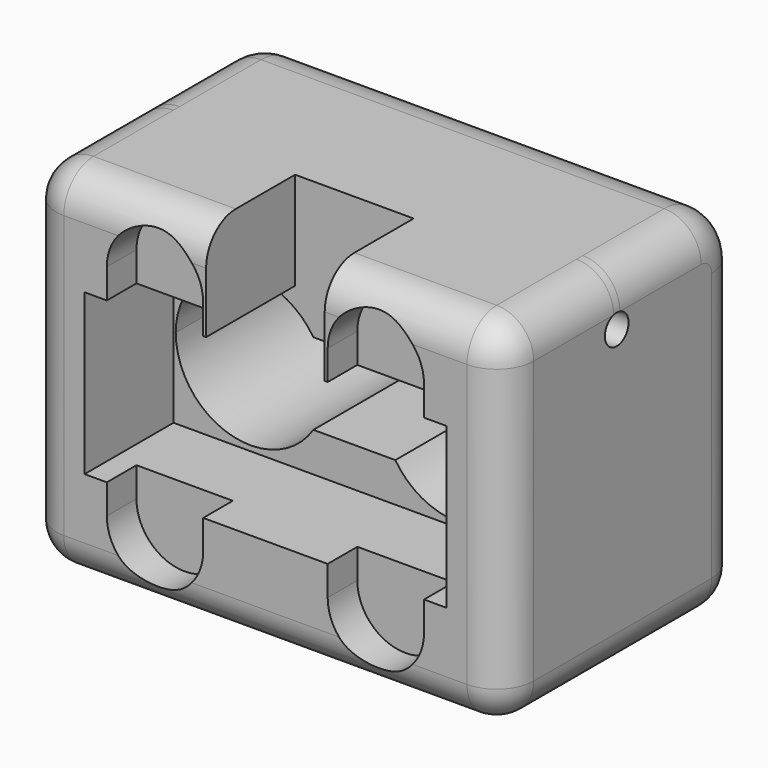
from build123d import *

# Parameters (mm, degrees)
F1_DEPTH      = 5
F3_DEPTH      = 10
F5_DEPTH      = 25
F7_R          = 6.7597979746
F6_R          = 2
F8_DEPTH      = 69.4
F9_R          = 5
F10_R         = 5
F11_T1_DEPTH  = 44.2
F11_T3_DEPTH  = 44.2
F12_T1_DEPTH  = 54.4
F12_T3_DEPTH  = 30
F12_T5_DEPTH  = 38
F12_S9_W      = 5
F12_S9_H      = 5
F12_T10_DEPTH = 5
F12_S15_W     = 5
F12_S15_H     = 5
F12_T16_DEPTH = 5
F12_S21_W     = 5
F12_S21_H     = 5
F12_T22_DEPTH = 5
F12_S27_W     = 5
F12_S27_H     = 5
F12_T28_DEPTH = 5
F12_T32_ANGLE = 90
F12_T34_ANGLE = 90


# Not quite as in the source:
# - a fillet or chamfer that OpenCascade refuses, or shapes differently, is made with other operations: its cross-section is extruded or revolved along the edge and cut away or added


with BuildPart() as f1:
    # F0 (on Front) → F1 (new body)
    with BuildSketch(Plane.XZ):
        with BuildLine():
            Line((32.2, -24), (32.2, 24))
            Line((32.2, 24), (8, 24))
            Line((8, 24), (8, 10.8))
            Line((8, 10.8), (8.4, 10.8))
            Line((8.4, 10.8), (8.4, 14.8))
            ThreePointArc((8.4, 14.8), (14.9, 21.3), (21.4, 14.8))
            Line((21.4, 14.8), (21.4, 10.8))
            Line((21.4, 10.8), (24.4, 10.8))
            Line((24.4, 10.8), (24.4, -10.8))
            Line((24.4, -10.8), (21.4, -10.8))
            Line((21.4, -10.8), (21.4, -14.8))
            ThreePointArc((21.4, -14.8), (14.9, -21.3), (8.4, -14.8))
            Line((8.4, -14.8), (8.4, -10.8))
            Line((8.4, -10.8), (-8.4, -10.8))
            Line((-8.4, -10.8), (-8.4, -14.8))
            ThreePointArc((-8.4, -14.8), (-14.9, -21.3), (-21.4, -14.8))
            Line((-21.4, -14.8), (-21.4, -10.8))
            Line((-21.4, -10.8), (-24.4, -10.8))
            Line((-24.4, -10.8), (-24.4, 10.8))
            Line((-24.4, 10.8), (-21.4, 10.8))
            Line((-21.4, 10.8), (-21.4, 14.8))
            ThreePointArc((-21.4, 14.8), (-14.9, 21.3), (-8.4, 14.8))
            Line((-8.4, 14.8), (-8.4, 10.8))
            Line((-8.4, 10.8), (-8, 10.8))
            Line((-8, 10.8), (-8, 24))
            Line((-8, 24), (-32.2, 24))
            Line((-32.2, 24), (-32.2, -24))
            Line((-32.2, -24), (32.2, -24))
        make_face()
    extrude(amount=F1_DEPTH)

    # F2 (on face) → F3 (join)
    with BuildSketch(Plane(origin=(0, 0, 0), x_dir=(-1, 0, 0), z_dir=(0, 1, 0))):
        with BuildLine():
            Line((24.4, 10.8), (24.4, -10.8))
            Line((24.4, -10.8), (21.4, -10.8))
            Line((21.4, -10.8), (21.4, -14.8))
            ThreePointArc((21.4, -14.8), (14.9, -21.3), (8.4, -14.8))
            Line((8.4, -14.8), (8.4, -10.8))
            Line((8.4, -10.8), (-8.4, -10.8))
            Line((-8.4, -10.8), (-8.4, -14.8))
            ThreePointArc((-8.4, -14.8), (-14.9, -21.3), (-21.4, -14.8))
            Line((-21.4, -14.8), (-21.4, -10.8))
            Line((-21.4, -10.8), (-24.4, -10.8))
            Line((-24.4, -10.8), (-24.4, 10.8))
            Line((-24.4, 10.8), (-21.4, 10.8))
            Line((-21.4, 10.8), (-21.4, 14.8))
            ThreePointArc((-21.4, 14.8), (-14.9, 21.3), (-8.4, 14.8))
            Line((-8.4, 14.8), (-8.4, 10.8))
            Line((-8.4, 10.8), (-8, 10.8))
            Line((-8, 10.8), (-8, 24))
            Line((-8, 24), (-32.2, 24))
            Line((-32.2, 24), (-32.2, -24))
            Line((-32.2, -24), (32.2, -24))
            Line((32.2, -24), (32.2, 24))
            Line((32.2, 24), (8, 24))
            Line((8, 24), (8, 10.8))
            Line((8, 10.8), (8.4, 10.8))
            Line((8.4, 10.8), (8.4, 14.8))
            ThreePointArc((8.4, 14.8), (14.9, 21.3), (21.4, 14.8))
            Line((21.4, 14.8), (21.4, 10.8))
            Line((21.4, 10.8), (24.4, 10.8))
        make_face()
        with BuildLine():
            Line((21.4, -14.8), (21.4, -10.8))
            Line((21.4, -10.8), (8.4, -10.8))
            Line((8.4, -10.8), (8.4, -14.8))
            ThreePointArc((8.4, -14.8), (14.9, -21.3), (21.4, -14.8))
        make_face()
        with BuildLine():
            Line((-8.4, -14.8), (-8.4, -10.8))
            Line((-8.4, -10.8), (-21.4, -10.8))
            Line((-21.4, -10.8), (-21.4, -14.8))
            ThreePointArc((-21.4, -14.8), (-14.9, -21.3), (-8.4, -14.8))
        make_face()
        with BuildLine():
            Line((8.4, 10.8), (21.4, 10.8))
            Line((21.4, 10.8), (21.4, 14.8))
            ThreePointArc((21.4, 14.8), (14.9, 21.3), (8.4, 14.8))
            Line((8.4, 14.8), (8.4, 10.8))
        make_face()
        with BuildLine():
            Line((-21.4, 10.8), (-8.4, 10.8))
            Line((-8.4, 10.8), (-8.4, 14.8))
            ThreePointArc((-8.4, 14.8), (-14.9, 21.3), (-21.4, 14.8))
            Line((-21.4, 14.8), (-21.4, 10.8))
        make_face()
    extrude(amount=F3_DEPTH)

    # F4 (on face) → F5 (join)
    with BuildSketch(Plane(origin=(0, 10, 0), x_dir=(-1, 0, 0), z_dir=(0, 1, 0))):
        Polygon((32.2, -24), (32.2, 24), (8, 24), (8, 10.8), (24.4, 10.8), (24.4, -10.8), (-24.4, -10.8), (-24.4, 10.8), (-8, 10.8), (-8, 24), (-32.2, 24), (-32.2, -24), align=None)
        Polygon((8, 10.8), (8, 24), (-8, 24), (-8, 10.8), (-24.4, 10.8), (-24.4, -10.8), (24.4, -10.8), (24.4, 10.8), align=None)
        with BuildLine():
            ThreePointArc((5.5288725662, 5.5), (16.8680666762, 9.6842239514), (24.1, 0))
            ThreePointArc((24.1, 0), (16.8680666762, -9.6842239514), (5.5288725662, -5.5))
            Line((5.5288725662, -5.5), (0, -5.5))
            Line((0, -5.5), (-5.5288725662, -5.5))
            ThreePointArc((-5.5288725662, -5.5), (-24.1, 0), (-5.5288725662, 5.5))
            Line((-5.5288725662, 5.5), (0, 5.5))
            Line((0, 5.5), (5.5288725662, 5.5))
        make_face(mode=Mode.SUBTRACT)
    extrude(amount=F5_DEPTH)

    # F7
    f7_edges = [f1.edges().sort_by_distance(p)[0] for p in [
        (0, 35, 24),
    ]]
    fillet(f7_edges, radius=F7_R)

    # F6 (on face) → F8 (cut)
    with BuildSketch(Plane(origin=(-32.2, 0, 0), x_dir=(0, -1, 0), z_dir=(-1, 0, 0))):
        with Locations((-14, 17.0717967697)):
            Circle(F6_R)
    extrude(amount=-F8_DEPTH, mode=Mode.SUBTRACT)

    # F9
    f9_edges = [f1.edges().sort_by_distance(p)[0] for p in [
        (32.2, 33.020101, 22.020101),
        (32.2, 35, -3.379899),
    ]]
    fillet(f9_edges, radius=F9_R)

    # F10
    f10_edges = [f1.edges().sort_by_distance(p)[0] for p in [
        (-32.2, 35, -3.379899),
    ]]
    fillet(f10_edges, radius=F10_R)

    # F11: fillet of radius 5 on 2 edges, made by hand

    # F11_s2 → F11_t1 (cut)
    with BuildSketch(Plane.YZ.offset(-39.7)):
        with BuildLine():
            ThreePointArc((-5, 19), (-3.5355339059, 22.5355339059), (0, 24))
            Line((0, 24), (-5, 24))
            Line((-5, 24), (-5, 19))
        make_face()
    extrude(amount=F11_T1_DEPTH, mode=Mode.SUBTRACT)

    # F11_s4 → F11_t3 (cut)
    with BuildSketch(Plane.YZ.offset(-4.5)):
        with BuildLine():
            ThreePointArc((-5, 19), (-3.5355339059, 22.5355339059), (0, 24))
            Line((0, 24), (-5, 24))
            Line((-5, 24), (-5, 19))
        make_face()
    extrude(amount=F11_T3_DEPTH, mode=Mode.SUBTRACT)

    # F12: fillet of radius 5 on 8 edges, made by hand

    # F12_s2 → F12_t1 (cut)
    with BuildSketch(Plane.YZ.offset(-27.2)):
        with BuildLine():
            ThreePointArc((30, -24), (33.5355339059, -22.5355339059), (35, -19))
            Line((35, -19), (35, -24))
            Line((35, -24), (30, -24))
        make_face()
        with BuildLine():
            ThreePointArc((-5, -19), (-3.5355339059, -22.5355339059), (0, -24))
            Line((0, -24), (-5, -24))
            Line((-5, -24), (-5, -19))
        make_face()
    extrude(amount=F12_T1_DEPTH, mode=Mode.SUBTRACT)

    # F12_s4 → F12_t3 (cut)
    with BuildSketch(Plane.XZ.offset(-30)):
        with BuildLine():
            ThreePointArc((-27.2, -24), (-30.7355339059, -22.5355339059), (-32.2, -19))
            Line((-32.2, -19), (-32.2, -24))
            Line((-32.2, -24), (-27.2, -24))
        make_face()
        with BuildLine():
            ThreePointArc((32.2, -19), (30.7355339059, -22.5355339059), (27.2, -24))
            Line((27.2, -24), (32.2, -24))
            Line((32.2, -24), (32.2, -19))
        make_face()
    extrude(amount=F12_T3_DEPTH, mode=Mode.SUBTRACT)

    # F12_s6 → F12_t5 (cut)
    with BuildSketch(Plane.XY.offset(-19)):
        with BuildLine():
            ThreePointArc((27.2, -5), (30.7355339059, -3.5355339059), (32.2, 0))
            Line((32.2, 0), (32.2, -5))
            Line((32.2, -5), (27.2, -5))
        make_face()
        with BuildLine():
            ThreePointArc((-27.2, -5), (-30.7355339059, -3.5355339059), (-32.2, 0))
            Line((-32.2, 0), (-32.2, -5))
            Line((-32.2, -5), (-27.2, -5))
        make_face()
    extrude(amount=F12_T5_DEPTH, mode=Mode.SUBTRACT)


with BuildPart() as f12_tool8:
    # F12_s9 → F12_t10 (new body)
    with BuildSketch(Plane.XZ):
        with Locations((-29.7, 21.5)):
            Rectangle(F12_S9_W, F12_S9_H)
    extrude(amount=F12_T10_DEPTH)

    # F12_s11 → F12_t12 (revolve, cut)
    with BuildSketch(Plane(origin=(-27.2, 0, 19), x_dir=(0.7071067812, 0, -0.7071067812), z_dir=(-0.7071067812, 0, -0.7071067812))):
        with BuildLine():
            ThreePointArc((0, -5), (5, 0), (0, 5))
            Line((0, 5), (0, -5))
        make_face()
    revolve(axis=Axis((-27.2, 0, 19), (0, -1, 0)), mode=Mode.SUBTRACT)


with BuildPart() as f1_1:
    add(f1.part)

    # F12_t7: cut F12_tool8
    add(f12_tool8.part, mode=Mode.SUBTRACT)


with BuildPart() as f12_tool14:
    # F12_s15 → F12_t16 (new body)
    with BuildSketch(Plane.XZ):
        with Locations((29.7, 21.5)):
            Rectangle(F12_S15_W, F12_S15_H)
    extrude(amount=F12_T16_DEPTH)

    # F12_s17 → F12_t18 (revolve, cut)
    with BuildSketch(Plane(origin=(27.2, 0, 19), x_dir=(-0.7071067812, 0, -0.7071067812), z_dir=(-0.7071067812, 0, 0.7071067812))):
        with BuildLine():
            ThreePointArc((0, -5), (5, 0), (0, 5))
            Line((0, 5), (0, -5))
        make_face()
    revolve(axis=Axis((27.2, 0, 19), (0, -1, 0)), mode=Mode.SUBTRACT)


with BuildPart() as f1_2:
    add(f1_1.part)

    # F12_t13: cut F12_tool14
    add(f12_tool14.part, mode=Mode.SUBTRACT)


with BuildPart() as f12_tool20:
    # F12_s21 → F12_t22 (new body)
    with BuildSketch(Plane.XZ):
        with Locations((-29.7, -21.5)):
            Rectangle(F12_S21_W, F12_S21_H)
    extrude(amount=F12_T22_DEPTH)

    # F12_s23 → F12_t24 (revolve, cut)
    with BuildSketch(Plane(origin=(-27.2, 0, -19), x_dir=(0.7071067812, 0, 0.7071067812), z_dir=(0.7071067812, 0, -0.7071067812))):
        with BuildLine():
            ThreePointArc((0, -5), (5, 0), (0, 5))
            Line((0, 5), (0, -5))
        make_face()
    revolve(axis=Axis((-27.2, 0, -19), (0, -1, 0)), mode=Mode.SUBTRACT)


with BuildPart() as f1_3:
    add(f1_2.part)

    # F12_t19: cut F12_tool20
    add(f12_tool20.part, mode=Mode.SUBTRACT)


with BuildPart() as f12_tool26:
    # F12_s27 → F12_t28 (new body)
    with BuildSketch(Plane.XZ):
        with Locations((29.7, -21.5)):
            Rectangle(F12_S27_W, F12_S27_H)
    extrude(amount=F12_T28_DEPTH)

    # F12_s29 → F12_t30 (revolve, cut)
    with BuildSketch(Plane(origin=(27.2, 0, -19), x_dir=(-0.7071067812, 0, 0.7071067812), z_dir=(0.7071067812, 0, 0.7071067812))):
        with BuildLine():
            ThreePointArc((0, -5), (5, 0), (0, 5))
            Line((0, 5), (0, -5))
        make_face()
    revolve(axis=Axis((27.2, 0, -19), (0, -1, 0)), mode=Mode.SUBTRACT)


with BuildPart() as f1_4:
    add(f1_3.part)

    # F12_t25: cut F12_tool26
    add(f12_tool26.part, mode=Mode.SUBTRACT)

    # F12_s31 → F12_t32 (revolve, cut)
    with BuildSketch(Plane.XZ.offset(-30)):
        with BuildLine():
            ThreePointArc((-27.2, -24), (-30.7355339059, -22.5355339059), (-32.2, -19))
            Line((-32.2, -19), (-32.2, -24))
            Line((-32.2, -24), (-27.2, -24))
        make_face()
    revolve(axis=Axis((-27.2, 30, -24), (0, 0, -1)), revolution_arc=F12_T32_ANGLE, mode=Mode.SUBTRACT)

    # F12_s33 → F12_t34 (revolve, cut)
    with BuildSketch(Plane.XZ.offset(-30)):
        with BuildLine():
            ThreePointArc((27.2, -24), (30.7355339059, -22.5355339059), (32.2, -19))
            Line((32.2, -19), (32.2, -24))
            Line((32.2, -24), (27.2, -24))
        make_face()
    revolve(axis=Axis((27.2, 30, -24), (0, 0, 1)), revolution_arc=F12_T34_ANGLE, mode=Mode.SUBTRACT)


solid = f1_4.part
